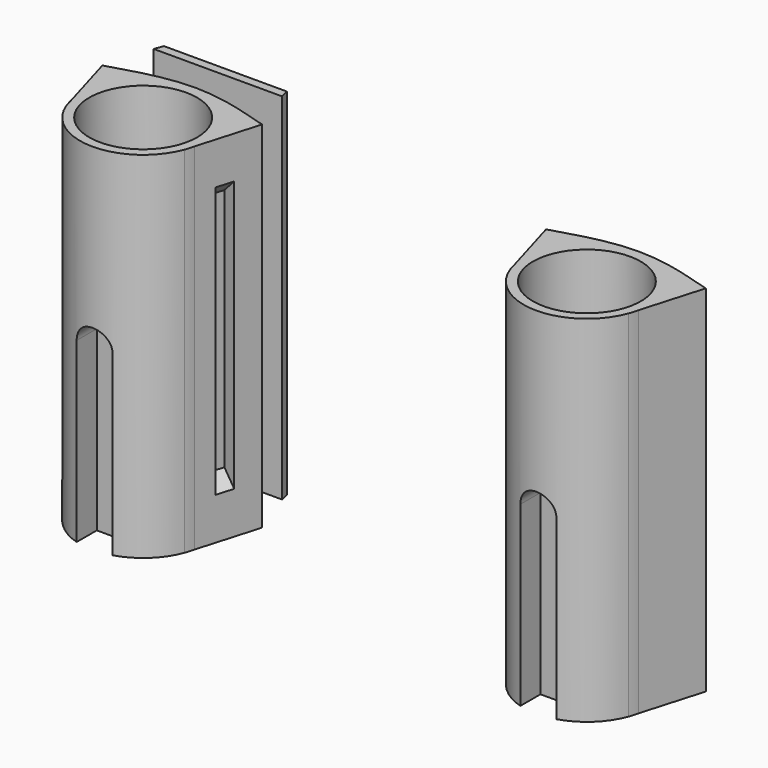
from build123d import *

# Parameters (mm, degrees)
F0_R        = 0.85
F1_DEPTH    = 40
F3_R        = 6.075
F4_DEPTH    = 14
F6_DEPTH    = 40
F9_DEPTH    = 6
F11_W       = 2
F11_H       = 30
F13_DEPTH   = 1
F12_W       = 2
F12_H       = 30.5
F14_DEPTH   = 1.5
F15_SIZE    = 0.99999
F16_SIZE2   = 0.1322452355
F16_SIZE    = 0.75
F16_2_SIZE2 = 0.1322452355
F16_2_SIZE  = 0.75
F17_SIZE    = 1.49999


# Not quite as in the source:
# - a fillet or chamfer is up to 0.001 mm smaller than in the source, because OpenCascade refuses the exact size


with BuildPart() as f1:
    # F0 (on Top) → F1 (new body)
    with BuildSketch(Plane.XY):
        with BuildLine():
            Line((-6.9716463271, -1.4702967352), (-6.6720030725, -2.5))
            ThreePointArc((-6.6720030725, -2.5), (0, -7.125), (6.6720030725, -2.5))
            Line((6.6720030725, -2.5), (6.9716463271, -1.4702967352))
            ThreePointArc((6.9716463271, -1.4702967352), (7.0865578767, -0.739136293), (7.125, 0))
            ThreePointArc((7.125, 0), (-0.739136293, 7.0865578767), (-6.9716463271, -1.4702967352))
        make_face()
        Circle(F0_R, mode=Mode.SUBTRACT)
        with BuildLine():
            ThreePointArc((-6.9716463271, -1.4702967352), (-6.8412253609, -1.9907939525), (-6.6720030725, -2.5))
            Line((-6.6720030725, -2.5), (-6.9716463271, -1.4702967352))
        make_face()
        with BuildLine():
            Line((6.9716463271, -1.4702967352), (6.6720030725, -2.5))
            ThreePointArc((6.6720030725, -2.5), (6.8412253609, -1.9907939525), (6.9716463271, -1.4702967352))
        make_face()
        with BuildLine():
            Line((-9, 5.5), (-6.9716463271, -1.4702967352))
            ThreePointArc((-6.9716463271, -1.4702967352), (-0.739136293, 7.0865578767), (7.125, 0))
            ThreePointArc((7.125, 0), (7.0865578767, -0.739136293), (6.9716463271, -1.4702967352))
            Line((6.9716463271, -1.4702967352), (9, 5.5))
            Line((9, 5.5), (6.9381416086, 6.1))
            add(Edge.make_bspline(
                [(0, 7.3087555656), (2.5162656326, 7.2960948201), (5.0063073264, 6.69804741), (6.9381416086, 6.1)],
                knots=[0.0229980904, 0.0229980904, 0.0229980904, 0.0229980904, 7.0669493094, 7.0669493094, 7.0669493094, 7.0669493094], degree=3))
            add(Edge.make_bspline(
                [(0, 7.3087555656), (-2.5162656326, 7.2960948201), (-5.0063073264, 6.69804741), (-6.9381416086, 6.1)],
                knots=[0.0229980904, 0.0229980904, 0.0229980904, 0.0229980904, 7.0669493094, 7.0669493094, 7.0669493094, 7.0669493094], degree=3))
            Line((-6.9381416086, 6.1), (-9, 5.5))
        make_face()
    extrude(amount=F1_DEPTH)

    # F3 (on face) → F4 (cut)
    with BuildSketch(Plane.XY.offset(40)):
        Circle(F3_R)
    extrude(amount=-F4_DEPTH, mode=Mode.SUBTRACT)

    # F8 (on offset) → F9 (cut)
    with BuildSketch(Plane.XZ.offset(10)):
        with BuildLine():
            Line((-2.0273134933, 20), (-2.0273134933, 0))
            Line((-2.0273134933, 0), (2.0273134933, 0))
            Line((2.0273134933, 0), (2.0273134933, 20))
            ThreePointArc((2.0273134933, 20), (0, 22.0273134933), (-2.0273134933, 20))
        make_face()
    extrude(amount=-F9_DEPTH, mode=Mode.SUBTRACT)


with BuildPart() as f6:
    # F5 (on Top) → F6 (new body)
    with BuildSketch(Plane.XY):
        Polygon((6.7794237824, 11.7658044089), (-7.0748599067, 11.7658044089), (-7.4343305431, 10.7781669524), (7.0256694569, 10.7781669524), align=None)
    extrude(amount=F6_DEPTH)


with BuildPart() as f10_1:
    # F10: instance of F1
    add(f1.part.mirror(Plane.YZ.offset(25)))

    # F11 (on face) → F13 (join)
    with BuildSketch(Plane(origin=(39.2746869048, 11.4289188052, 0), x_dir=(0.2794096775, -0.9601719805, 0), z_dir=(-0.9601719805, -0.2794096775, 0))):
        with Locations((10.1748508868, 20)):
            Rectangle(F11_W, F11_H)
    extrude(amount=F13_DEPTH)

    # F15 (size 1 in the source; OpenCascade refuses exactly that, so slightly less here)
    f15_edges = [f10_1.edges().sort_by_distance(p)[0] for p in [
        (41.157467, 1.379902, 5),
        (41.157467, 1.379902, 35),
    ]]
    chamfer(f15_edges, length=F15_SIZE)

    # F16
    f16_edges = [f10_1.edges().sort_by_distance(p)[0] for p in [
        (41.436876, 0.41973, 20),
    ]]
    f16_side = f10_1.faces().sort_by_distance((41.922481, 0.561041, 20))[0]
    chamfer(f16_edges, length=F16_SIZE, length2=F16_SIZE2, reference=f16_side)

    # F16#2
    f16_2_edges = [f10_1.edges().sort_by_distance(p)[0] for p in [
        (40.878057, 2.340074, 20),
    ]]
    f16_2_side = f10_1.faces().sort_by_distance((41.363661, 2.481385, 20))[0]
    chamfer(f16_2_edges, length=F16_2_SIZE, length2=F16_2_SIZE2, reference=f16_2_side)


with BuildPart() as f1_1:
    add(f1.part)

    # F12 (on face) → F14 (cut)
    with BuildSketch(Plane(origin=(6.8218246998, -1.9851483676, 0), x_dir=(0.2794096775, 0.9601719805, 0), z_dir=(0.9601719805, -0.2794096775, 0))):
        with Locations((3.7956329906, 20)):
            Rectangle(F12_W, F12_H)
    extrude(amount=-F14_DEPTH, mode=Mode.SUBTRACT)

    # F17 (size 1.5 in the source; OpenCascade refuses exactly that, so slightly less here)
    f17_edges = [f1_1.edges().sort_by_distance(p)[0] for p in [
        (6.442103, 2.078427, 35.25),
        (6.442103, 2.078427, 4.75),
    ]]
    chamfer(f17_edges, length=F17_SIZE)


solid = Compound([f6.part, f10_1.part, f1_1.part])
